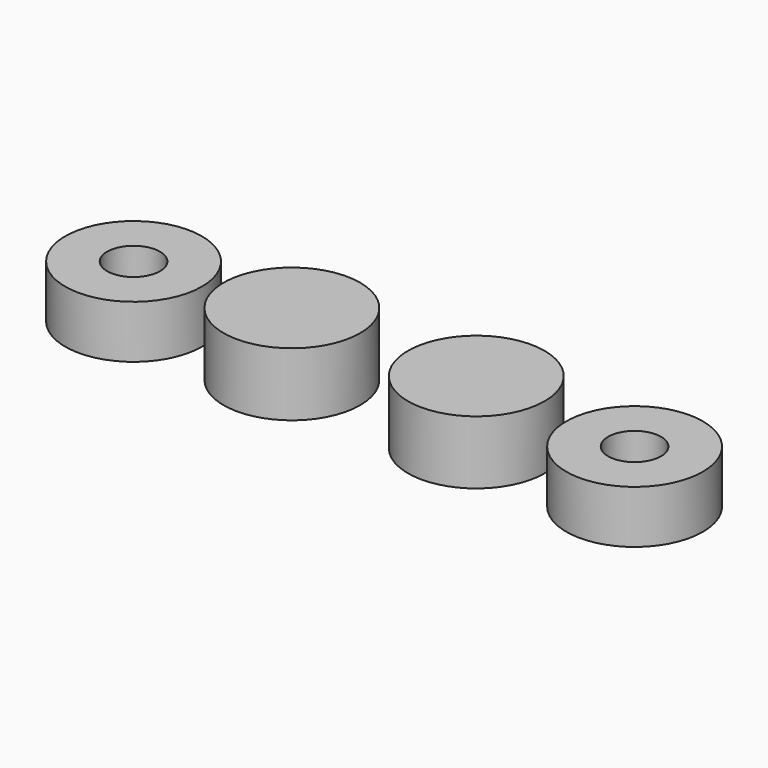
from build123d import *

# Parameters (mm, degrees)
F0_R     = 10.25
F1_DEPTH = 9.525
F0_R_2   = 3.96875
F2_DEPTH = 7.9375


# Not quite as in the source:
# - a length typed as a fraction of an inch, garbled in the dataset ("3 / 203.2 mm" for 3/8 in), is restored
# - a feature names something its author has since deleted; it is built from what else it names


with BuildPart() as f1:
    # F0 (on Top) → F1 (new body)
    with BuildSketch(Plane.XY):
        Circle(F0_R)
    extrude(amount=F1_DEPTH)


with BuildPart() as f1b:
    # F0 (on Top) → F1, piece 2 (new body)
    with BuildSketch(Plane.XY):
        with Locations((-27.6688113809, 0)):
            Circle(F0_R)
    extrude(amount=F1_DEPTH)


with BuildPart() as f2:
    # F0 (on Top) → F2 (new body)
    with BuildSketch(Plane.XY):
        with Locations((-51.425293088, 0)):
            Circle(F0_R)
        with Locations((-51.425293088, 0)):
            Circle(F0_R_2, mode=Mode.SUBTRACT)
    extrude(amount=F2_DEPTH)


with BuildPart() as f2b:
    # F0 (on Top) → F2, piece 2 (new body)
    with BuildSketch(Plane.XY):
        with Locations((23.7564817071, 0)):
            Circle(F0_R)
        with Locations((23.7564817071, 0)):
            Circle(F0_R_2, mode=Mode.SUBTRACT)
    extrude(amount=F2_DEPTH)


solid = Compound([f1.part, f1b.part, f2.part, f2b.part])
